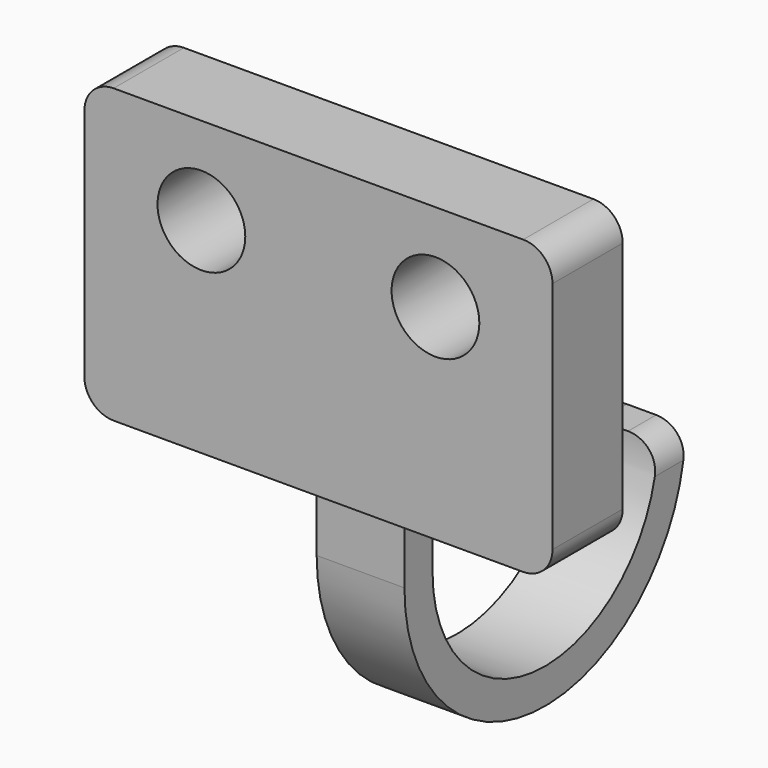
from build123d import *

# Parameters (mm, degrees)
F1_DEPTH    = 19.05
F2_R        = 6.35
F0_W        = 19.05
F0_H        = 19.05
F3_DEPTH    = 7.62
F4_W        = 19.05
F4_H        = 7.62
F5_ANGLE    = 180
F6_T1_DEPTH = 39.37
F7_R        = 9.525
F8_DEPTH    = 19.051
F9_R        = 9.525
F10_DEPTH   = 12.7


# Not quite as in the source:
# - a fillet or chamfer that OpenCascade refuses, or shapes differently, is made with other operations: its cross-section is extruded or revolved along the edge and cut away or added


with BuildPart() as f1:
    # F0 (on Front) → F1 (new body)
    with BuildSketch(Plane.XZ):
        Polygon((50.8, -31.75), (50.8, 31.75), (-50.8, 31.75), (-50.8, -31.75), (-9.525, -31.75), (9.525, -31.75), align=None)
    extrude(amount=F1_DEPTH)

    # F2
    f2_edges = [f1.edges().sort_by_distance(p)[0] for p in [
        (50.8, -9.525, 31.75),
        (50.8, -9.525, -31.75),
        (-50.8, -9.525, -31.75),
        (-50.8, -9.525, 31.75),
    ]]
    fillet(f2_edges, radius=F2_R)

    # F0 (on Front) → F3 (join)
    with BuildSketch(Plane.XZ):
        with Locations((0, -41.275)):
            Rectangle(F0_W, F0_H)
    extrude(amount=F3_DEPTH)

    # F4 (on face) → F5 (revolve)
    with BuildSketch(Plane(origin=(0, 0, -50.8), x_dir=(1, 0, 0), z_dir=(0, 0, -1))):
        with Locations((0, 3.81)):
            Rectangle(F4_W, F4_H)
    revolve(axis=Axis((-4.1156476188, 30.4856614615, -50.8), (1, 0, 0)), revolution_arc=F5_ANGLE)

    # F6: fillet of radius 6.35 on 3 edges, made by hand

    # F6_s2 → F6_t1 (cut)
    with BuildSketch(Plane.XZ.offset(-84.4663229229)):
        with BuildLine():
            ThreePointArc((-9.525, -57.15), (-7.6651280605, -52.6598719395), (-3.175, -50.8))
            Line((-3.175, -50.8), (-9.525, -50.8))
            Line((-9.525, -50.8), (-9.525, -57.15))
        make_face()
        with BuildLine():
            ThreePointArc((9.525, -57.15), (7.6651280605, -52.6598719395), (3.175, -50.8))
            Line((3.175, -50.8), (9.525, -50.8))
            Line((9.525, -50.8), (9.525, -57.15))
        make_face()
    extrude(amount=F6_T1_DEPTH, mode=Mode.SUBTRACT)

    # F7 (on face) → F8 (cut, through all)
    with BuildSketch(Plane.XZ):
        with Locations((-25.4, 12.7)):
            Circle(F7_R)
        with Locations((25.4, 12.7)):
            Circle(F7_R)
    extrude(amount=F8_DEPTH, mode=Mode.SUBTRACT)

    # F9 (on face) → F10 (cut)
    with BuildSketch(Plane.XZ):
        with Locations((0, -6.35)):
            Circle(F9_R)
    extrude(amount=F10_DEPTH, mode=Mode.SUBTRACT)


solid = f1.part
